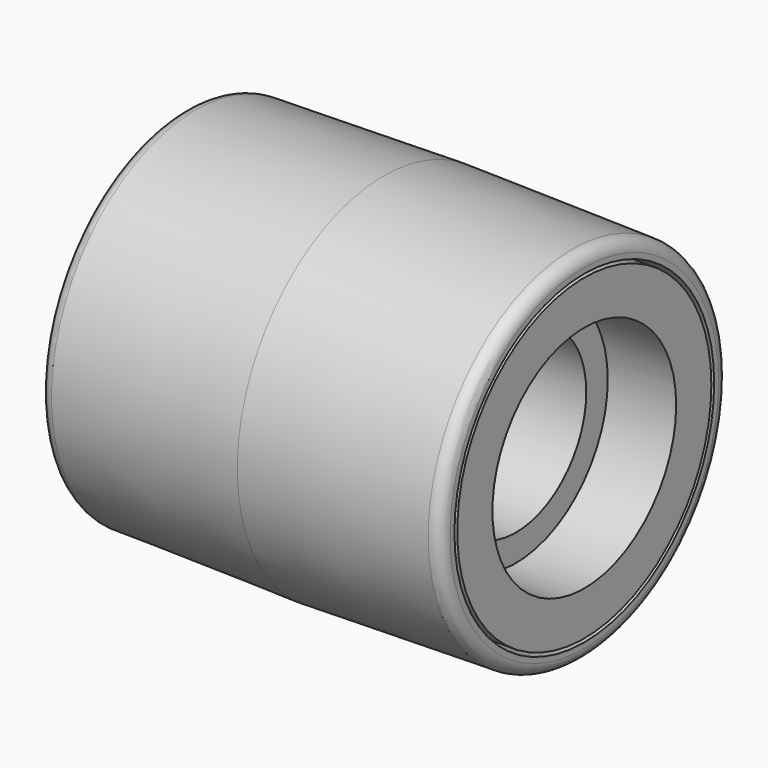
from build123d import *

# Parameters (mm, degrees)
F0_R          = 37.5
F0_R_2        = 32.5
F1_DEPTH      = 41
F1_TAPER      = 1
F2_R          = 2.5
F3_DEPTH      = 41
F4_R          = 23.5
F5_DEPTH      = 14
F7_R          = 18
F8_DEPTH      = 27
F8_DEPTH_BACK = 27


with BuildPart() as f1:
    # F0 (on Right) → F1 (new body, symmetric)
    with BuildSketch(Plane.YZ):
        Circle(F0_R)
        Circle(F0_R_2, mode=Mode.SUBTRACT)
    extrude(amount=F1_DEPTH, both=True, taper=F1_TAPER)

    # F2
    f2_edges = [f1.edges().sort_by_distance(p)[0] for p in [
        (41, -36.784342, 0),
        (-41, -36.784342, 0),
    ]]
    fillet(f2_edges, radius=F2_R)


with BuildPart() as f3:
    # F0 (on Right) → F3 (new body, symmetric)
    with BuildSketch(Plane.YZ):
        Circle(F0_R_2)
    extrude(amount=F3_DEPTH, both=True)

    # F4 (on face) → F5 (cut)
    with BuildSketch(Plane.YZ.offset(41)):
        Circle(F4_R)
    f5 = extrude(amount=-F5_DEPTH, mode=Mode.SUBTRACT)

    # F6: F5 across plane
    add(f5.mirror(Plane.YZ), mode=Mode.SUBTRACT)

    # F7 (on Right) → F8 (cut, two sides)
    with BuildSketch(Plane.YZ) as f8_sk:
        Circle(F7_R)
    extrude(amount=-F8_DEPTH, mode=Mode.SUBTRACT)
    extrude(f8_sk.sketch, amount=F8_DEPTH_BACK, mode=Mode.SUBTRACT)


solid = Compound([f1.part, f3.part])
